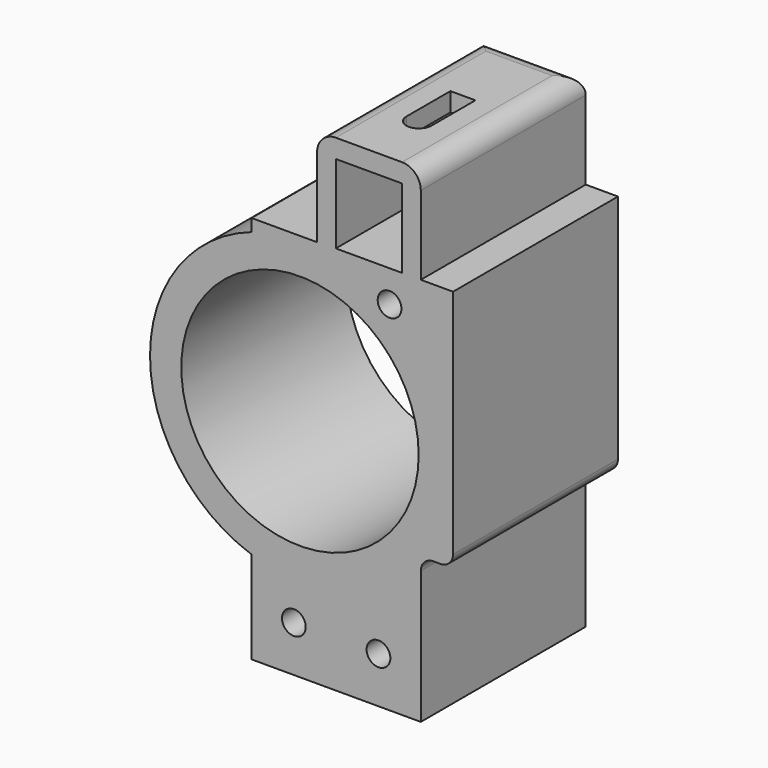
from build123d import *

# Parameters (mm, degrees)
F0_R      = 1.9
F0_R_2    = 19
F1_DEPTH  = 33
F2_W      = 10.6
F2_H      = 12.6
F3_DEPTH  = 6.7
F4_R      = 3
F5_R      = 2
F7_DEPTH  = 8.5
F8_R      = 1.99999
F9_R      = 2.15
F9_R_2    = 1
F10_DEPTH = 3
F11_DEPTH = 3.5


# Not quite as in the source:
# - a fillet or chamfer is up to 0.001 mm smaller than in the source, because OpenCascade refuses the exact size


with BuildPart() as f1:
    # F0 (on Front) → F1 (new body)
    with BuildSketch(Plane.XZ):
        with BuildLine():
            Line((-109.659200659, 0), (-109.659200659, 10.3))
            Line((-109.659200659, 10.3), (-126.259200659, 10.3))
            Line((-126.259200659, 10.3), (-126.259200659, 0))
            Line((-126.259200659, 0), (-126.259200659, -5))
            Line((-126.259200659, -5), (-126.259200659, -5.4))
            Line((-126.259200659, -5.4), (-136.75, -5.4))
            Line((-136.75, -5.4), (-136.75, -7.385742363))
            ThreePointArc((-136.75, -7.385742363), (-153, -30.1), (-136.75, -52.814257637))
            Line((-136.75, -52.814257637), (-136.75, -67.6))
            Line((-136.75, -67.6), (-132.812420773, -67.6))
            Line((-132.812420773, -67.6), (-109.659200659, -67.6))
            Line((-109.659200659, -67.6), (-109.659200659, -44.3103300754))
            Line((-109.659200659, -44.3103300754), (-105, -44.3103300754))
            Line((-105, -44.3103300754), (-104.5, -44.3103300754))
            Line((-104.5, -44.3103300754), (-104.5, -5.3))
            Line((-104.5, -5.3), (-105, -5.3))
            Line((-105, -5.3), (-109.659200659, -5.3))
            Line((-109.659200659, -5.3), (-109.659200659, 0))
        make_face()
        with Locations((-129.9773001648, -60.2071288185)):
            Circle(F0_R, mode=Mode.SUBTRACT)
        with Locations((-129, -30.1)):
            Circle(F0_R_2, mode=Mode.SUBTRACT)
        with Locations((-116.4319004943, -60.2071288185)):
            Circle(F0_R, mode=Mode.SUBTRACT)
        with Locations((-114.659200659, -10.3896699246)):
            Circle(F0_R, mode=Mode.SUBTRACT)
        Polygon((-112.659200659, -5.3), (-117.959200659, -5.3), (-123.259200659, -5.3), (-123.259200659, 7.3), (-112.659200659, 7.3), align=None, mode=Mode.SUBTRACT)
    extrude(amount=F1_DEPTH)

    # F2 (on face) → F3 (join)
    with BuildSketch(Plane(origin=(0, 0, 0), x_dir=(-1, 0, 0), z_dir=(0, 1, 0))):
        with Locations((117.959200659, 1)):
            Rectangle(F2_W, F2_H)
    extrude(amount=-F3_DEPTH)

    # F4
    f4_edges = [f1.edges().sort_by_distance(p)[0] for p in [
        (-109.659201, -16.5, 10.3),
        (-126.259201, -16.5, 10.3),
        (-117.959201, 0, 10.3),
    ]]
    fillet(f4_edges, radius=F4_R)

    # F5
    f5_edges = [f1.edges().sort_by_distance(p)[0] for p in [
        (-104.5, -16.5, -44.31033),
        (-109.659201, -16.5, -44.31033),
    ]]
    fillet(f5_edges, radius=F5_R)

    # F6 (on face) → F7 (cut)
    with BuildSketch(Plane.XY.offset(10.3)):
        Polygon((-119.959200659, -25), (-117.959200659, -25), (-115.959200659, -25), (-115.959200659, -14.2), (-119.959200659, -14.2), align=None)
    extrude(amount=-F7_DEPTH, mode=Mode.SUBTRACT)

    # F8 (radius 2 in the source; OpenCascade refuses exactly that, so slightly less here)
    f8_edges = [f1.edges().sort_by_distance(p)[0] for p in [
        (-119.959201, -25, 8.8),
        (-115.959201, -25, 8.8),
    ]]
    fillet(f8_edges, radius=F8_R)

    # F9 (on face) → F10 (cut)
    with BuildSketch(Plane.XZ.offset(6.7)):
        with Locations((-117.959200659, 1)):
            Circle(F9_R)
        with Locations((-117.959200659, 1)):
            Circle(F9_R_2, mode=Mode.SUBTRACT)
    extrude(amount=-F10_DEPTH, mode=Mode.SUBTRACT)

    # F11 (add): a face of the model
    f11_faces = [f1.faces().sort_by_distance(p)[0] for p in [
        (-117.959200659, -6.7, 1),
    ]]
    extrude(f11_faces, amount=F11_DEPTH)


solid = f1.part
